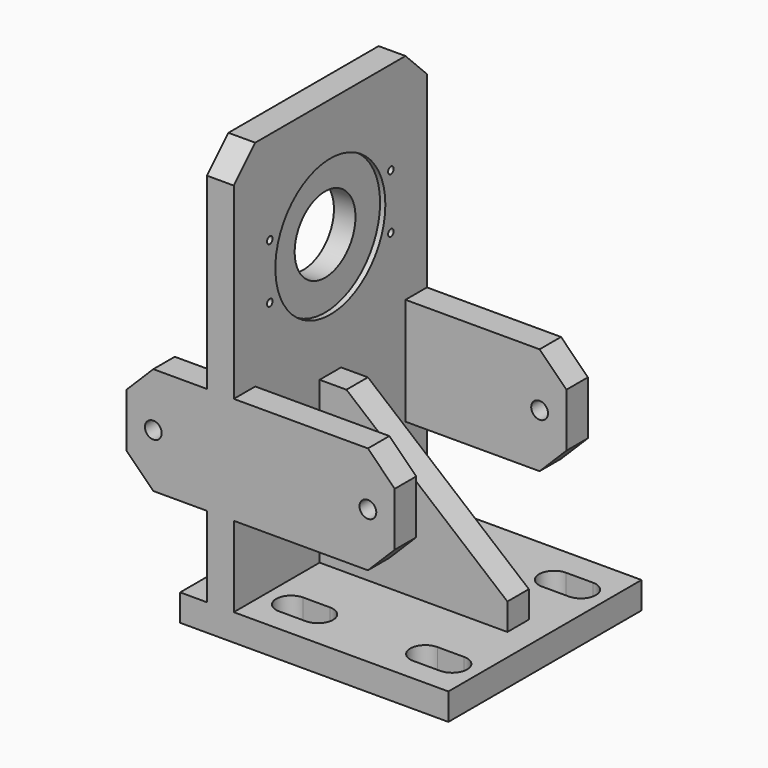
from build123d import *

# Parameters (mm, degrees)
F0_W           = 127
F0_H           = 114.3
F1_DEPTH       = 12.7
F2_W           = 12.7
F2_H           = 114.3
F3_DEPTH       = 190.5
F4_SIZE        = 12.7
F6_D           = 36
F6_CBORE_D     = 65.1
F6_CBORE_DEPTH = 2.5
F8_D           = 3.3
F8_DEPTH       = 10
F8_TIP         = 0.9914200214
F9_W           = 38.1
F9_H           = 50.8
F10_DEPTH      = 12.7
F9_W_2         = 76.2
F11_SIZE       = 12.7
F11_2_SIZE     = 12.7
F13_D          = 7.9375
F13_2_D        = 7.9375
F15_W          = 88.9
F15_H          = 12.7
F16_DEPTH      = 76.2
F17_SIZE2      = 76.2
F17_SIZE       = 63.5


# Not quite as in the source:
# - a length typed as a fraction of an inch, garbled in the dataset ("3 / 203.2 mm" for 3/8 in), is restored


with BuildPart() as f1:
    # F0 (on Top) → F1 (new body)
    with BuildSketch(Plane.XY):
        Rectangle(F0_W, F0_H)
        with BuildLine():
            ThreePointArc((-25.4, -46.1646754677), (-32.512, -39.0526754677), (-25.4, -31.9406754677))
            Line((-25.4, -31.9406754677), (-12.7, -31.9406754677))
            ThreePointArc((-12.7, -31.9406754677), (-5.588, -39.0526754677), (-12.7, -46.1646754677))
            Line((-12.7, -46.1646754677), (-25.4, -46.1646754677))
        make_face(mode=Mode.SUBTRACT)
        with BuildLine():
            ThreePointArc((38.1, -46.1646754677), (30.988, -39.0526754677), (38.1, -31.9406754677))
            Line((38.1, -31.9406754677), (50.8, -31.9406754677))
            ThreePointArc((50.8, -31.9406754677), (57.912, -39.0526754677), (50.8, -46.1646754677))
            Line((50.8, -46.1646754677), (38.1, -46.1646754677))
        make_face(mode=Mode.SUBTRACT)
        with BuildLine():
            ThreePointArc((-25.4, 30.0353245323), (-32.512, 37.1473245323), (-25.4, 44.2593245323))
            Line((-25.4, 44.2593245323), (-12.7, 44.2593245323))
            ThreePointArc((-12.7, 44.2593245323), (-5.588, 37.1473245323), (-12.7, 30.0353245323))
            Line((-12.7, 30.0353245323), (-25.4, 30.0353245323))
        make_face(mode=Mode.SUBTRACT)
        with BuildLine():
            Line((50.8, 30.0353245323), (38.1, 30.0353245323))
            ThreePointArc((38.1, 30.0353245323), (30.988, 37.1473245323), (38.1, 44.2593245323))
            Line((38.1, 44.2593245323), (50.8, 44.2593245323))
            ThreePointArc((50.8, 44.2593245323), (57.912, 37.1473245323), (50.8, 30.0353245323))
        make_face(mode=Mode.SUBTRACT)
    extrude(amount=F1_DEPTH)

    # F2 (on face) → F3 (join)
    with BuildSketch(Plane.XY.offset(12.7)):
        with Locations((-44.45, 0)):
            Rectangle(F2_W, F2_H)
    extrude(amount=F3_DEPTH)

    # F4
    f4_edges = [f1.edges().sort_by_distance(p)[0] for p in [
        (-44.45, 57.15, 203.2),
        (-44.45, -57.15, 203.2),
    ]]
    chamfer(f4_edges, length=F4_SIZE)

    # F6 (through all)
    with Locations(Plane.YZ.offset(-38.1)):
        with Locations((0, 146.05)):
            CounterBoreHole(F6_D / 2, F6_CBORE_D / 2, F6_CBORE_DEPTH)

    # F8
    with Locations(Plane.YZ.offset(-38.1)):
        with Locations((-35.814, 159.08522997), (-35.814, 133.01477003), (35.814, 133.01477003), (35.814, 159.08522997)):
            Hole(F8_D / 2, depth=F8_DEPTH)
            with Locations((0, 0, -(F8_DEPTH + F8_TIP / 2))):  # 118° drill point
                Cone(0, F8_D / 2, F8_TIP, mode=Mode.SUBTRACT)



with BuildPart() as f10:
    # F9 (on face) → F10 (new body)
    with BuildSketch(Plane.XZ.offset(57.15)):
        with Locations((-69.85, 76.2)):
            Rectangle(F9_W, F9_H)
    extrude(amount=-F10_DEPTH)

    # F11
    f11_edges = [f10.edges().sort_by_distance(p)[0] for p in [
        (-88.9, -50.8, 101.6),
        (-88.9, -50.8, 50.8),
    ]]
    chamfer(f11_edges, length=F11_SIZE)

    # F13 (through all)
    with Locations(Plane.XZ.offset(57.15)):
        with Locations((-76.2, 76.2), (25.4, 76.2)):
            Hole(F13_D / 2)


with BuildPart() as f10b:
    # F9 (on face) → F10, piece 2 (new body)
    with BuildSketch(Plane.XZ.offset(57.15)):
        with Locations((0, 76.2)):
            Rectangle(F9_W_2, F9_H)
    extrude(amount=-F10_DEPTH)

    # F11#2
    f11_2_edges = [f10b.edges().sort_by_distance(p)[0] for p in [
        (38.1, -50.8, 101.6),
        (38.1, -50.8, 50.8),
    ]]
    chamfer(f11_2_edges, length=F11_2_SIZE)

    # F13#2 (through all)
    with Locations(Plane.XZ.offset(57.15)):
        with Locations((-76.2, 76.2), (25.4, 76.2)):
            Hole(F13_2_D / 2)


with BuildPart() as f1_1:
    add(f1.part)

    add(f10.part)  # F14 merges F10

    add(f10b.part)  # F14 merges F10b
    # F14: F10b, F10 across plane
    add(f10b.part.mirror(Plane.XZ))
    add(f10.part.mirror(Plane.XZ))

    # F15 (on face) → F16 (join)
    with BuildSketch(Plane.XY.offset(12.7)):
        with Locations((6.35, 0)):
            Rectangle(F15_W, F15_H)
    extrude(amount=F16_DEPTH)

    # F17
    f17_edges = [f1_1.edges().sort_by_distance(p)[0] for p in [
        (50.8, 0, 88.9),
    ]]
    f17_side = f1_1.faces().sort_by_distance((50.8, 0, 50.8))[0]
    chamfer(f17_edges, length=F17_SIZE, length2=F17_SIZE2, reference=f17_side)


solid = f1_1.part
